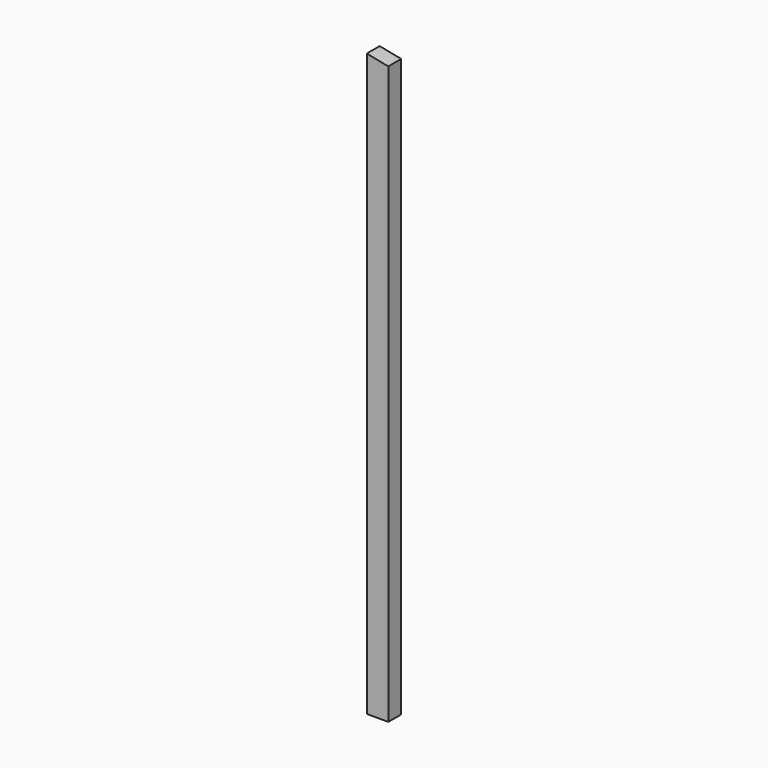
from build123d import *

# Parameters (mm, degrees)
F0_W     = 100
F0_H     = 75
F1_DEPTH = 2700
F2_SIZE2 = 19.981962
F2_SIZE  = 99.99999


# Not quite as in the source:
# - a fillet or chamfer is up to 0.001 mm smaller than in the source, because OpenCascade refuses the exact size


with BuildPart() as f1:
    # F0 (on Top) → F1 (new body)
    with BuildSketch(Plane.XY):
        with Locations((-39.2657851032, 37.5)):
            Rectangle(F0_W, F0_H)
    extrude(amount=F1_DEPTH)

    # F2 (size 100 and 19.9819717699 in the source; OpenCascade refuses exactly that, so slightly less here)
    f2_edges = [f1.edges().sort_by_distance(p)[0] for p in [
        (10.734215, 37.5, 2700),
    ]]
    f2_side = f1.faces().sort_by_distance((-39.265785, 37.5, 2700))[0]
    chamfer(f2_edges, length=F2_SIZE, length2=F2_SIZE2, reference=f2_side)


solid = f1.part
